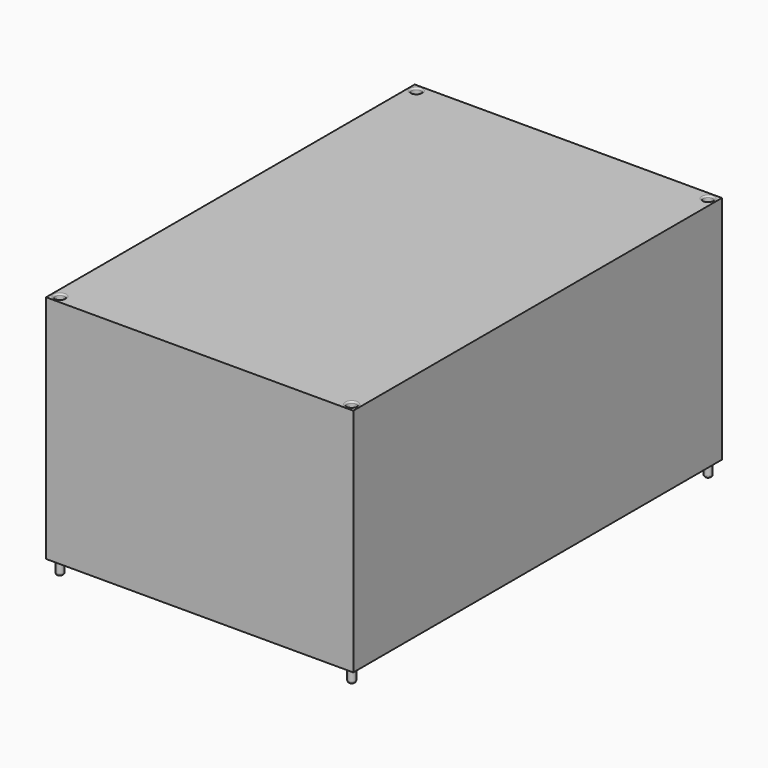
from build123d import *

# Parameters (mm, degrees)
F0_W     = 101.6
F0_H     = 152.4
F0_R     = 1.5875
F0_W_2   = 91.44
F0_H_2   = 142.24
F1_DEPTH = 6.35
F2_DEPTH = 69.85
F3_R     = 1.190625
F4_DEPTH = 4.7625
F5_R     = 0.762
F6_R     = 0.508


# Not quite as in the source:
# - a length typed as a fraction of an inch, garbled in the dataset ("3 / 203.2 mm" for 3/8 in), is restored


with BuildPart() as f1:
    # F0 (on Top) → F1 (new body)
    with BuildSketch(Plane.XY):
        Rectangle(F0_W, F0_H)
        with Locations((-48.26, -73.66)):
            Circle(F0_R, mode=Mode.SUBTRACT)
        with Locations((48.26, -73.66)):
            Circle(F0_R, mode=Mode.SUBTRACT)
        Rectangle(F0_W_2, F0_H_2, mode=Mode.SUBTRACT)
        with Locations((-48.26, 73.66)):
            Circle(F0_R, mode=Mode.SUBTRACT)
        with Locations((48.26, 73.66)):
            Circle(F0_R, mode=Mode.SUBTRACT)
        Rectangle(F0_W_2, F0_H_2)
    extrude(amount=F1_DEPTH)

    # F0 (on Top) → F2 (join)
    with BuildSketch(Plane.XY):
        Rectangle(F0_W, F0_H)
        with Locations((-48.26, -73.66)):
            Circle(F0_R, mode=Mode.SUBTRACT)
        with Locations((48.26, -73.66)):
            Circle(F0_R, mode=Mode.SUBTRACT)
        Rectangle(F0_W_2, F0_H_2, mode=Mode.SUBTRACT)
        with Locations((-48.26, 73.66)):
            Circle(F0_R, mode=Mode.SUBTRACT)
        with Locations((48.26, 73.66)):
            Circle(F0_R, mode=Mode.SUBTRACT)
        with Locations((48.26, -73.66)):
            Circle(F0_R)
        with Locations((-48.26, -73.66)):
            Circle(F0_R)
        with Locations((-48.26, 73.66)):
            Circle(F0_R)
        with Locations((48.26, 73.66)):
            Circle(F0_R)
    extrude(amount=-F2_DEPTH)

    # F3 (on face) → F4 (join)
    with BuildSketch(Plane(origin=(0, 0, -69.85), x_dir=(1, 0, 0), z_dir=(0, 0, -1))):
        with Locations((48.26, 73.66)):
            Circle(F3_R)
        with Locations((48.26, -73.66)):
            Circle(F3_R)
        with Locations((-48.26, -73.66)):
            Circle(F3_R)
        with Locations((-48.26, 73.66)):
            Circle(F3_R)
    extrude(amount=F4_DEPTH)

    # F5
    f5_edges = [f1.edges().sort_by_distance(p)[0] for p in [
        (47.069375, -73.66, -74.6125),
        (-49.450625, -73.66, -74.6125),
        (-49.450625, 73.66, -74.6125),
        (47.069375, 73.66, -74.6125),
    ]]
    fillet(f5_edges, radius=F5_R)

    # F6
    f6_edges = [f1.edges().sort_by_distance(p)[0] for p in [
        (-49.8475, -73.66, 6.35),
        (-49.8475, 73.66, 6.35),
        (46.6725, 73.66, 6.35),
        (46.6725, -73.66, 6.35),
    ]]
    fillet(f6_edges, radius=F6_R)


solid = f1.part
